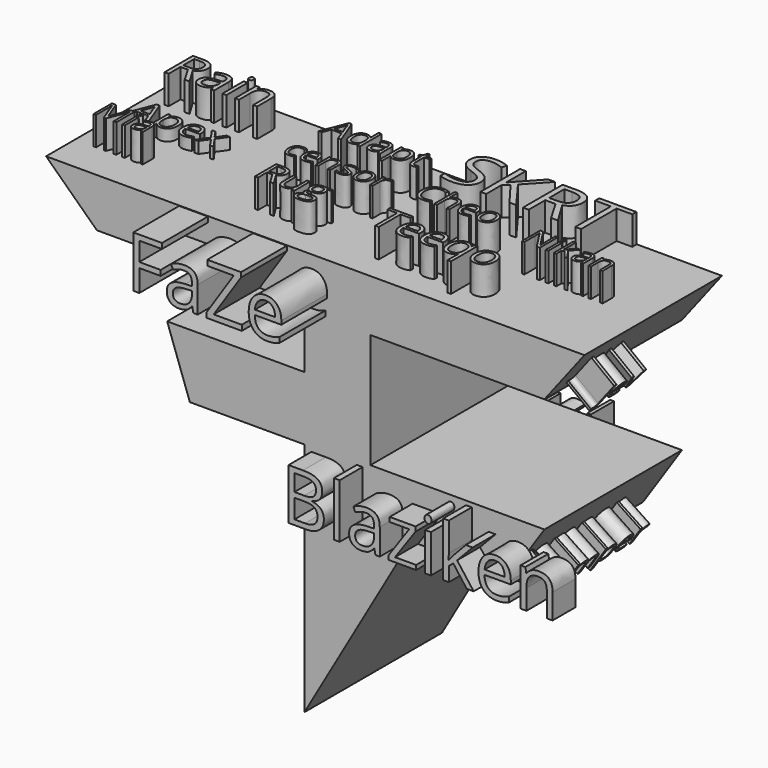
from build123d import *

# Parameters (mm, degrees)
F1_DEPTH      = 38.1
F2_DEPTH      = 25.4
F3_TEXT_SIZE  = 15.9748411183
F4_DEPTH      = 12.7
F5_TEXT_SIZE  = 11.0336883356
F6_DEPTH      = 6.35
F7_TEXT_SIZE  = 8.6693274271
F8_DEPTH      = 2.54
F9_TEXT_SIZE  = 7.8812053996
F10_DEPTH     = 6.35
F11_TEXT_SIZE = 7.0930872526
F12_DEPTH     = 6.35
F13_TEXT_SIZE = 15.8239788481
F14_DEPTH     = 6.35
F15_TEXT_SIZE = 15.3683514024
F16_DEPTH     = 6.35
F17_TEXT_SIZE = 7.4871440625
F18_DEPTH     = 6.35
F19_TEXT_SIZE = 7.0930846656
F20_DEPTH     = 6.35
F21_TEXT_SIZE = 8.2752641497
F22_DEPTH     = 6.35
F23_TEXT_SIZE = 9.4574462208
F24_DEPTH     = 6.35
F25_TEXT_SIZE = 7.0930872526
F26_DEPTH     = 6.35
F27_TEXT_SIZE = 10.0904923966
F28_DEPTH     = 6.35
F29_TEXT_SIZE = 11.2934891755
F30_DEPTH     = 6.35
F31_TEXT_SIZE = 8.189215076
F32_DEPTH     = 6.35
F33_TEXT_SIZE = 8.1058798565
F34_DEPTH     = 6.35


# Not quite as in the source:
# - Text() gives the source's letters only with a copy of the font that has no kerning and outlines rounded to 1/6400 em; it was checked with that copy


with BuildPart() as f1:
    # F0 (on Front) → F1 (new body)
    with BuildSketch(Plane.XZ):
        Polygon((58.5877349141, 49.8415084842), (-52.8367921115, 49.8415084842), (-60.7443361054, 49.8415084842), (-49.4820749523, 39.0584899427), (-3.4745270256, 39.0584899427), (-3.4745270256, 26.3584899427), (-33.9066027644, 26.3584899427), (-28.8745270256, 12.2207542421), (-3.4745270256, 12.2207542421), (-3.4745270256, -40.0169814586), (19.5292449714, 0), (41.0952820542, 0), (49.7216962581, 12.939622879), (11.1424520733, 12.939622879), (11.1424520733, 38.339622879), (49.7216962581, 38.339622879), align=None)
    extrude(amount=F1_DEPTH)

    # F0 (on Front) → F2 (join)
    with BuildSketch(Plane.XZ):
        Polygon((58.5877349141, 49.8415084842), (-52.8367921115, 49.8415084842), (-60.7443361054, 49.8415084842), (-49.4820749523, 39.0584899427), (-3.4745270256, 39.0584899427), (-3.4745270256, 26.3584899427), (-33.9066027644, 26.3584899427), (-28.8745270256, 12.2207542421), (-3.4745270256, 12.2207542421), (-3.4745270256, -40.0169814586), (19.5292449714, 0), (41.0952820542, 0), (49.7216962581, 12.939622879), (11.1424520733, 12.939622879), (11.1424520733, 38.339622879), (49.7216962581, 38.339622879), align=None)
    extrude(amount=F2_DEPTH)

    # F3 (on face) → F4 (join)
    with BuildSketch(Plane.XZ.offset(38.1)):
        with Locations((-32.811768353, 38.339622879)):
            Text('FaZe', F3_TEXT_SIZE, font='Open Sans', text_align=(TextAlign.LEFT, TextAlign.BOTTOM))
    extrude(amount=F4_DEPTH)

    # F5 (on face) → F6 (join)
    with BuildSketch(Plane.XY.offset(49.8415084842)):
        with Locations((-57.8795745969, -10.2140428498)):
            Text('Rain', F5_TEXT_SIZE, font='Open Sans', text_align=(TextAlign.LEFT, TextAlign.BOTTOM))
    extrude(amount=F6_DEPTH)

    # F7 (on face) → F8 (join)
    with BuildSketch(Plane.XY.offset(49.8415084842)):
        with Locations((-57.3121272027, -20.9955330938)):
            Text('Apex', F7_TEXT_SIZE, font='Open Sans', text_align=(TextAlign.LEFT, TextAlign.BOTTOM))
    extrude(amount=F8_DEPTH)

    # F9 (on face) → F10 (join)
    with BuildSketch(Plane.XY.offset(49.8415084842)):
        with Locations((-22.157270118, -10.7814893126)):
            Text('Adapt', F9_TEXT_SIZE, font='Open Sans', text_align=(TextAlign.LEFT, TextAlign.BOTTOM))
    extrude(amount=F10_DEPTH)

    # F11 (on face) → F12 (join)
    with BuildSketch(Plane.XY.offset(49.8415084842)):
        with Locations((-22.6335981052, -20.9955330938)):
            Text('censor', F11_TEXT_SIZE, font='Open Sans', text_align=(TextAlign.LEFT, TextAlign.BOTTOM))
    extrude(amount=F12_DEPTH)

    # F13 (on face) → F14 (join)
    with BuildSketch(Plane.XZ.offset(38.1)):
        with Locations((-3.4745270256, 0)):
            Text('Blaziken', F13_TEXT_SIZE, font='Open Sans', text_align=(TextAlign.LEFT, TextAlign.BOTTOM))
    extrude(amount=F14_DEPTH)

    # F15 (on face) → F16 (join)
    with BuildSketch(Plane.XY.offset(49.8415084842)):
        with Locations((3.9721284993, -11.0652130097)):
            Text('SKRT', F15_TEXT_SIZE, font='Open Sans', text_align=(TextAlign.LEFT, TextAlign.BOTTOM))
    extrude(amount=F16_DEPTH)

    # F17 (on face) → F18 (join)
    with BuildSketch(Plane.XY.offset(49.8415084842)):
        with Locations((5.1070218906, -19.5769146085)):
            Text('Cheo', F17_TEXT_SIZE, font='Open Sans', text_align=(TextAlign.LEFT, TextAlign.BOTTOM))
    extrude(amount=F18_DEPTH)

    # F19 (on face) → F20 (join)
    with BuildSketch(Plane.XY.offset(49.8415084842)):
        with Locations((-57.3121272027, -30.0746820867)):
            Text('Mia', F19_TEXT_SIZE, font='Open Sans', text_align=(TextAlign.LEFT, TextAlign.BOTTOM))
    extrude(amount=F20_DEPTH)

    # F21 (on face) → F22 (join)
    with BuildSketch(Plane.XY.offset(49.8415084842)):
        with Locations((-20.9955330938, -30.9258513153)):
            Text('Rug', F21_TEXT_SIZE, font='Open Sans', text_align=(TextAlign.LEFT, TextAlign.BOTTOM))
    extrude(amount=F22_DEPTH)

    # F23 (on face) → F24 (join)
    with BuildSketch(Plane.XY.offset(49.8415084842)):
        with Locations((5.390746519, -32.3444679379)):
            Text('Teeqo', F23_TEXT_SIZE, font='Open Sans', text_align=(TextAlign.LEFT, TextAlign.BOTTOM))
    extrude(amount=F24_DEPTH)

    # F25 (on face) → F26 (join)
    with BuildSketch(Plane.XY.offset(49.8415084842)):
        with Locations((30.3584057838, -20.9955330938)):
            Text('Nikan', F25_TEXT_SIZE, font='Open Sans', text_align=(TextAlign.LEFT, TextAlign.BOTTOM))
    extrude(amount=F26_DEPTH)

    # F27 (on face) → F28 (join)
    with BuildSketch(Plane(origin=(0, 0, 0), x_dir=(-1, 0, 0), z_dir=(0, 1, 0))):
        with Locations((-30.4320741657, 5.6744683534)):
            Text('banks', F27_TEXT_SIZE, font='Open Sans', text_align=(TextAlign.LEFT, TextAlign.BOTTOM))
    extrude(amount=F28_DEPTH)

    # F29 (on face) → F30 (join)
    with BuildSketch(Plane(origin=(-21.767137146, 0, -7.7476255785), x_dir=(0, -1, 0), z_dir=(-0.942102625, 0, -0.3353246845))):
        with Locations((1.986066578, 24.7875470668)):
            Text('Milan', F29_TEXT_SIZE, font='Open Sans', text_align=(TextAlign.LEFT, TextAlign.BOTTOM))
    extrude(amount=F30_DEPTH)

    # F31 (on face) → F32 (join)
    with BuildSketch(Plane(origin=(28.4505820122, 0, -18.9670523689), x_dir=(0, 1, 0), z_dir=(0.8320503255, 0, -0.5547001495))):
        with Locations((-38.1, 26.2054912746)):
            Text('temper', F31_TEXT_SIZE, font='Open Sans', text_align=(TextAlign.LEFT, TextAlign.BOTTOM))
    extrude(amount=F32_DEPTH)

    # F33 (on face) → F34 (join)
    with BuildSketch(Plane(origin=(12.6511289627, 0, -9.7519139275), x_dir=(0, 1, 0), z_dir=(0.7920101361, 0, -0.6105079396))):
        with Locations((-33.4700830281, 64.9442374706)):
            Text('Jev', F33_TEXT_SIZE, font='Open Sans', text_align=(TextAlign.LEFT, TextAlign.BOTTOM))
    extrude(amount=F34_DEPTH)


solid = f1.part
